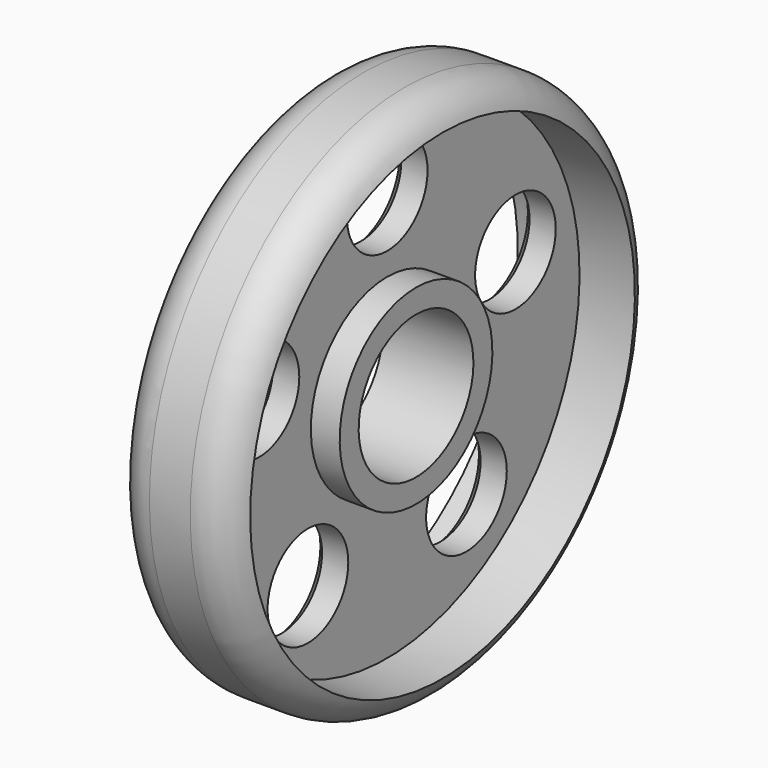
from build123d import *

# Parameters (mm, degrees)
F2_R     = 6.2570278464
F3_DEPTH = 25
F5_SIZE  = 1


# Not quite as in the source:
# - a fillet or chamfer that OpenCascade refuses, or shapes differently, is made with other operations: its cross-section is extruded or revolved along the edge and cut away or added


with BuildPart() as f1:
    # F0 (on Front) → F1 (revolve)
    with BuildSketch(Plane.XZ):
        Polygon((0, 11.8446564302), (0, 8.9004915208), (11.2406639382, 8.9004915208), (11.2406639382, 11.8446564302), (7.6611181721, 11.8446564302), (7.6611181721, 29.8391282558), (14.5299769938, 29.8391282558), (14.5299769938, 33.2251861691), (0, 33.2251861691), (0, 29.8391282558), (3.4043616615, 29.8391282558), (3.4043616615, 11.8446564302), align=None)
    revolve(axis=Axis((7.4493242428, 0, 0), (1, 0, 0)))

    # F2 (on face) → F3 (cut)
    with BuildSketch(Plane.YZ.offset(7.6611181721)):
        with Locations((0, 20.9185741842)):
            Circle(F2_R)
        with Locations((19.8947462895, 6.464194921)):
            Circle(F2_R)
        with Locations((12.2956294044, -16.9234820131)):
            Circle(F2_R)
        with Locations((-12.2956294044, -16.9234820131)):
            Circle(F2_R)
        with Locations((-19.8947462895, 6.464194921)):
            Circle(F2_R)
    extrude(amount=-F3_DEPTH, mode=Mode.SUBTRACT)

    # F4: fillet of radius 5 on 3 edges, made by hand

    # F4_s1 → F4_t2 (revolve, cut)
    with BuildSketch(Plane.XZ):
        with BuildLine():
            ThreePointArc((9.7976212442, 33.2251861691), (12.7071134307, 32.2914934887), (14.5299769938, 29.8391282558))
            Line((14.5299769938, 29.8391282558), (14.6246241088, 29.8714070976))
            ThreePointArc((14.6246241088, 29.8714070976), (14.6299769938, 31.5321572125), (14.6299769938, 33.2251861691))
            Line((14.6299769938, 33.2251861691), (14.5299769938, 33.3251861691))
            Line((14.5299769938, 33.3251861691), (9.7976212442, 33.3251861691))
            Line((9.7976212442, 33.3251861691), (9.7976212442, 33.2251861691))
        make_face()
    revolve(axis=Axis((14.5299769938, 0, 0), (1, 0, 0)), mode=Mode.SUBTRACT)

    # F4_s3 → F4_t4 (revolve, cut)
    with BuildSketch(Plane.XZ):
        with BuildLine():
            ThreePointArc((0, 29.8391282558), (1.8228635631, 32.2914934887), (4.7323557496, 33.2251861691))
            Line((4.7323557496, 33.2251861691), (4.7323557496, 33.3251861691))
            Line((4.7323557496, 33.3251861691), (0, 33.3251861691))
            Line((0, 33.3251861691), (-0.1, 33.2251861691))
            ThreePointArc((-0.1, 33.2251861691), (-0.1, 31.5321572125), (-0.094647115, 29.8714070976))
            Line((-0.094647115, 29.8714070976), (0, 29.8391282558))
        make_face()
    revolve(axis=Axis((0, 0, 0), (1, 0, 0)), mode=Mode.SUBTRACT)

    # F5
    f5_edges = [f1.edges().sort_by_distance(p)[0] for p in [
        (3.404362, -6.257028, 20.918574),
        (3.404362, -26.151774, 6.464195),
        (3.404362, -18.552657, -16.923482),
        (3.404362, 6.038602, -16.923482),
        (3.404362, 13.637718, 6.464195),
    ]]
    chamfer(f5_edges, length=F5_SIZE)


solid = f1.part
